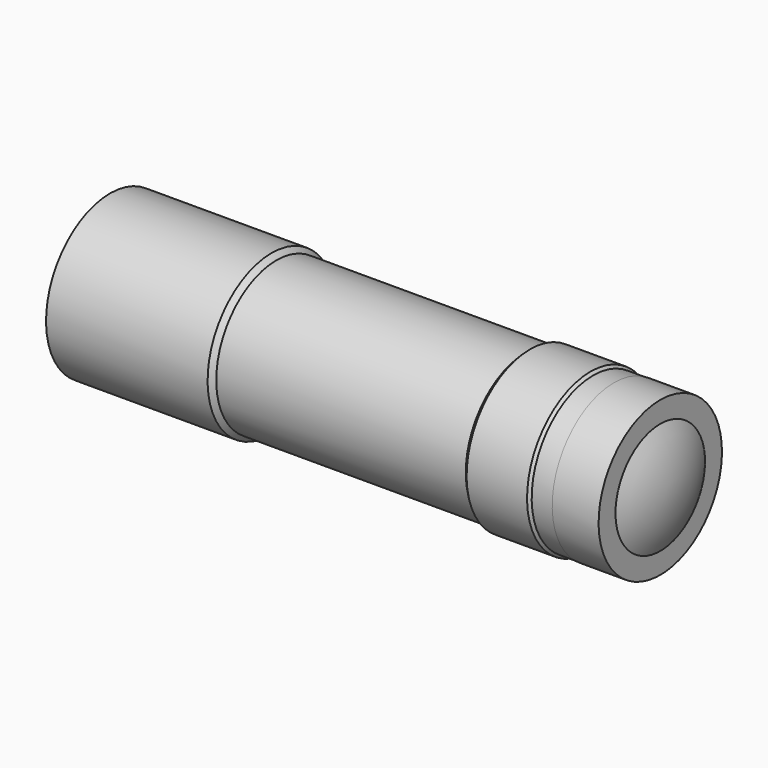
from build123d import *

# Parameters (mm, degrees)
F2_SIZE = 0.74999
F3_SIZE = 0.64999
F4_SIZE = 0.39999


# Not quite as in the source:
# - a fillet or chamfer is up to 0.001 mm smaller than in the source, because OpenCascade refuses the exact size


with BuildPart() as f1:
    # F0 (on Front) → F1 (revolve)
    with BuildSketch(Plane.XZ):
        with BuildLine():
            Line((-85.55, 11.75), (-85.55, 0))
            Line((-85.55, 0), (0, 0))
            ThreePointArc((0, 0), (-0.5715031948, 4.5173277499), (-2.25, 8.75))
            Line((-2.25, 8.75), (-2.25, 12.05))
            Line((-2.25, 12.05), (-9.5, 12.05))
            Line((-9.5, 12.05), (-9.5, 12))
            Line((-9.5, 12), (-12.75, 12))
            Line((-12.75, 12), (-12.75, 12.4))
            Line((-12.75, 12.4), (-23.25, 12.4))
            Line((-23.25, 12.4), (-23.25, 11.75))
            Line((-23.25, 11.75), (-62.25, 11.75))
            Line((-62.25, 11.75), (-62.25, 12.5))
            Line((-62.25, 12.5), (-88.25, 12.5))
            Line((-88.25, 12.5), (-88.25, 11.75))
            Line((-88.25, 11.75), (-85.55, 11.75))
        make_face()
    revolve(axis=Axis((-46.3619604707, 0, 0), (-1, 0, 0)))

    # F2 (size 0.75 in the source; OpenCascade refuses exactly that, so slightly less here)
    f2_edges = [f1.edges().sort_by_distance(p)[0] for p in [
        (-62.25, 0, -12.5),
    ]]
    chamfer(f2_edges, length=F2_SIZE)

    # F3 (size 0.65 in the source; OpenCascade refuses exactly that, so slightly less here)
    f3_edges = [f1.edges().sort_by_distance(p)[0] for p in [
        (-23.25, 0, -12.4),
    ]]
    chamfer(f3_edges, length=F3_SIZE)

    # F4 (size 0.4 in the source; OpenCascade refuses exactly that, so slightly less here)
    f4_edges = [f1.edges().sort_by_distance(p)[0] for p in [
        (-12.75, 0, -12.4),
    ]]
    chamfer(f4_edges, length=F4_SIZE)


solid = f1.part
